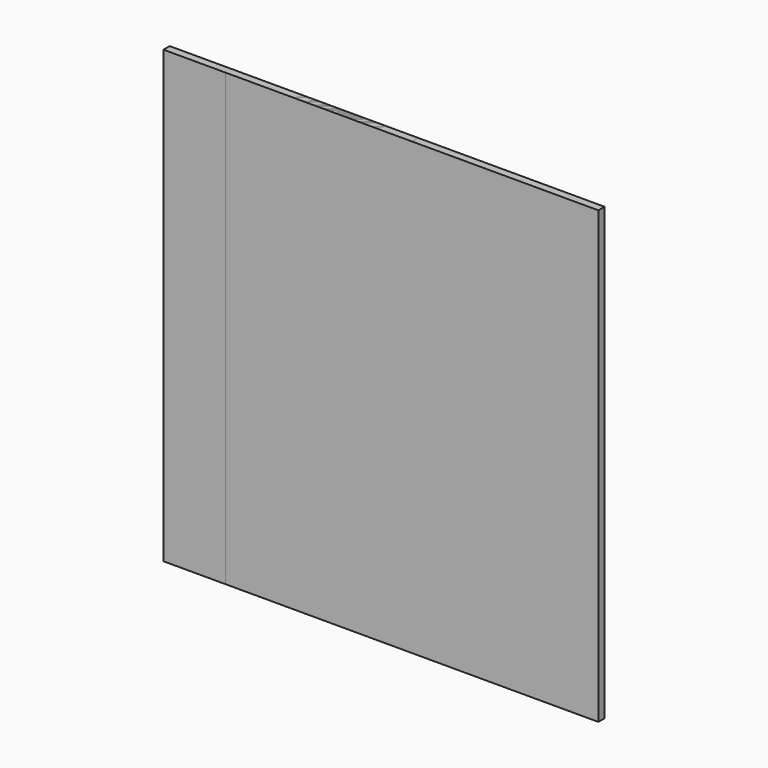
from build123d import *

# Parameters (mm, degrees)
F1_DEPTH      = 3.175
F3_START      = -12.7
F2_W          = 5.08
F2_H          = 5.08
F2_R          = 1.5875
F3_DEPTH      = 31.75
F5_DEPTH      = 44.45
F5_DEPTH_BACK = 12.7


# Not quite as in the source:
# - ends of sketch curves that miss each other by under 0.0002 mm in the source are joined
# - a feature names something its author has since deleted; it is built from what else it names


with BuildPart() as f1:
    # F0 (on Front) → F1 (new body)
    with BuildSketch(Plane.XZ):
        Polygon((98.6998776882, -152.6810299752), (128.3797776882, -152.6810299752), (128.3797776882, -78.3310389752), (98.6998768725, -78.3310389752), (98.6998769073, -81.5060299752), (125.2047776882, -81.5060299752), (125.2047776882, -149.5060299752), (98.6998776534, -149.5060299752), align=None)
        Polygon((174.8998776882, -152.6810299752), (174.8998776882, 31.4689700248), (98.6998756677, 31.4689700248), (98.6998768725, -78.3310389752), (128.3797776882, -78.3310389752), (128.3797776882, -152.6810299752), align=None)
        Polygon((125.2047776882, -81.5060299752), (98.6998769073, -81.5060299752), (98.6998776534, -149.5060299752), (125.2047776882, -149.5060299752), align=None)
    extrude(amount=F1_DEPTH)

    # F2 (on face) → F3 (join)
    with BuildSketch(Plane.YZ.offset(174.8998776882).offset(F3_START)):
        with Locations((2.54, 16.2289700248)):
            Rectangle(F2_W, F2_H)
        with Locations((2.54, 16.2289700248)):
            Circle(F2_R, mode=Mode.SUBTRACT)
        with Locations((2.54, -99.3410299752)):
            Rectangle(F2_W, F2_H)
        with Locations((2.54, -99.3410299752)):
            Circle(F2_R, mode=Mode.SUBTRACT)
    extrude(amount=-F3_DEPTH)

    # F4: F1 across face


with BuildPart() as f1_1:
    add(f1.part)
    add(f1.part.mirror(Plane(origin=(98.699876678, -1.5875, -60.6060299752), x_dir=(0, -1, 0), z_dir=(-1, 0, -1.1e-08))))


with BuildPart() as f5:
    # F2 (on face) → F5 (new body, two sides)
    with BuildSketch(Plane.YZ.offset(174.8998776882)) as f5_sk:
        with Locations((2.54, 16.2289700248)):
            Circle(F2_R)
    extrude(amount=-F5_DEPTH)
    extrude(f5_sk.sketch, amount=F5_DEPTH_BACK)


with BuildPart() as f5b:
    # F2 (on face) → F5, piece 2 (new body, two sides)
    with BuildSketch(Plane.YZ.offset(174.8998776882)) as f5_2_sk:
        with Locations((2.54, -99.3410299752)):
            Circle(F2_R)
    extrude(amount=-F5_DEPTH)
    extrude(f5_2_sk.sketch, amount=F5_DEPTH_BACK)


with BuildPart() as f7_1:
    # F7: instance of F1
    add(f1_1.part.mirror(Plane(origin=(111.3998739817, 2.54, 16.2289703035), x_dir=(0, 1, 0), z_dir=(1, 0, 2.19e-08))))


with BuildPart() as f7_2:
    # F7: instance of F5
    add(f5.part.mirror(Plane(origin=(111.3998739817, 2.54, 16.2289703035), x_dir=(0, 1, 0), z_dir=(1, 0, 2.19e-08))))


with BuildPart() as f7_3:
    # F7: instance of F5b
    add(f5b.part.mirror(Plane(origin=(111.3998739817, 2.54, 16.2289703035), x_dir=(0, 1, 0), z_dir=(1, 0, 2.19e-08))))


solid = Compound([f1_1.part, f5.part, f5b.part, f7_1.part, f7_2.part, f7_3.part])
